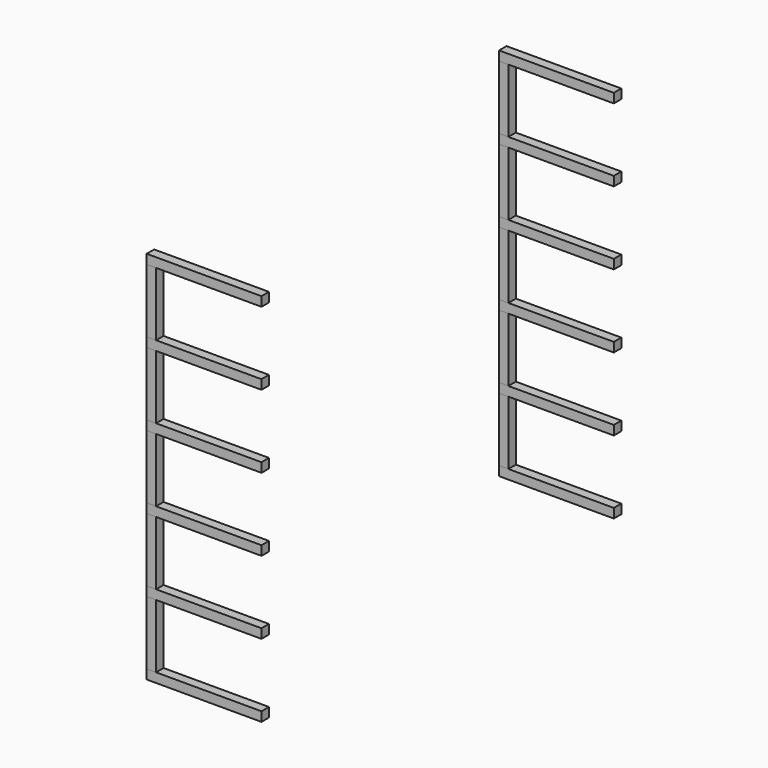
from build123d import *

# Parameters (mm, degrees)
F0_W     = 25.4
F0_H     = 25.4
F1_DEPTH = 311.15
F0_H_2   = 172.72
F2_DEPTH = 25.4
F3_DEPTH = 25.4
F4_DEPTH = 311.15


with BuildPart() as f1:
    # F0 (on Right) → F1 (new body)
    with BuildSketch(Plane.YZ):
        with Locations((-799.7573850555, 127.6102497262)):
            Rectangle(F0_W, F0_H)
    extrude(amount=F1_DEPTH)


with BuildPart() as f1b:
    # F0 (on Right) → F1, piece 2 (new body)
    with BuildSketch(Plane.YZ):
        with Locations((-799.7573850555, -466.7497502738)):
            Rectangle(F0_W, F0_H)
    extrude(amount=F1_DEPTH)


with BuildPart() as f1c:
    # F0 (on Right) → F1, piece 3 (new body)
    with BuildSketch(Plane.YZ):
        with Locations((-799.7573850555, 325.7302497262)):
            Rectangle(F0_W, F0_H)
    extrude(amount=F1_DEPTH)


with BuildPart() as f1d:
    # F0 (on Right) → F1, piece 4 (new body)
    with BuildSketch(Plane.YZ):
        with Locations((-799.7573850555, -268.6297502738)):
            Rectangle(F0_W, F0_H)
    extrude(amount=F1_DEPTH)


with BuildPart() as f1e:
    # F0 (on Right) → F1, piece 5 (new body)
    with BuildSketch(Plane.YZ):
        with Locations((-799.7573850555, -70.5097502738)):
            Rectangle(F0_W, F0_H)
    extrude(amount=F1_DEPTH)


with BuildPart() as f1f:
    # F0 (on Right) → F1, piece 6 (new body)
    with BuildSketch(Plane.YZ):
        with Locations((-799.7573850555, 523.8502497262)):
            Rectangle(F0_W, F0_H)
    extrude(amount=F1_DEPTH)


with BuildPart() as f2:
    # F0 (on Right) → F2 (new body)
    with BuildSketch(Plane.YZ):
        with Locations((-799.7573850555, -169.5697502738)):
            Rectangle(F0_W, F0_H_2)
    extrude(amount=F2_DEPTH)


with BuildPart() as f2b:
    # F0 (on Right) → F2, piece 2 (new body)
    with BuildSketch(Plane.YZ):
        with Locations((-799.7573850555, 226.6702497262)):
            Rectangle(F0_W, F0_H_2)
    extrude(amount=F2_DEPTH)


with BuildPart() as f2c:
    # F0 (on Right) → F2, piece 3 (new body)
    with BuildSketch(Plane.YZ):
        with Locations((-799.7573850555, 424.7902497262)):
            Rectangle(F0_W, F0_H_2)
    extrude(amount=F2_DEPTH)


with BuildPart() as f2d:
    # F0 (on Right) → F2, piece 4 (new body)
    with BuildSketch(Plane.YZ):
        with Locations((-799.7573850555, 28.5502497262)):
            Rectangle(F0_W, F0_H_2)
    extrude(amount=F2_DEPTH)


with BuildPart() as f2e:
    # F0 (on Right) → F2, piece 5 (new body)
    with BuildSketch(Plane.YZ):
        Polygon((-812.4573850555, -454.0497502738), (-787.0573850555, -454.0497502738), (-787.0573850555, -296.3315248489), (-787.0573850555, -281.3297502738), (-812.4573850555, -281.3297502738), (-812.4573850555, -296.3315248489), align=None)
    extrude(amount=F2_DEPTH)


with BuildPart() as f3:
    # F0 (on Right) → F3 (new body)
    with BuildSketch(Plane.YZ):
        Polygon((381.3426149445, -57.8097502738), (406.7426149445, -57.8097502738), (406.7426149445, 100.4313870019), (406.7426149445, 114.9102497262), (381.3426149445, 114.9102497262), align=None)
    extrude(amount=F3_DEPTH)


with BuildPart() as f3b:
    # F0 (on Right) → F3, piece 2 (new body)
    with BuildSketch(Plane.YZ):
        Polygon((381.3426149445, -255.9297502738), (406.7426149445, -255.9297502738), (406.7426149445, -83.2097502738), (393.4404167575, -83.2097502738), (381.3426149445, -83.2097502738), align=None)
    extrude(amount=F3_DEPTH)


with BuildPart() as f3c:
    # F0 (on Right) → F3, piece 3 (new body)
    with BuildSketch(Plane.YZ):
        with Locations((394.0426149445, 424.7902497262)):
            Rectangle(F0_W, F0_H_2)
    extrude(amount=F3_DEPTH)


with BuildPart() as f3d:
    # F0 (on Right) → F3, piece 4 (new body)
    with BuildSketch(Plane.YZ):
        Polygon((381.3426149445, -454.0497502738), (406.7426149445, -454.0497502738), (406.7426149445, -281.3297502738), (381.8395647449, -281.3297502738), (381.3426149445, -281.3297502738), align=None)
    extrude(amount=F3_DEPTH)


with BuildPart() as f3e:
    # F0 (on Right) → F3, piece 5 (new body)
    with BuildSketch(Plane.YZ):
        Polygon((381.3426149445, 140.3102497262), (406.7426149445, 140.3102497262), (406.7426149445, 313.0302497262), (395.5076758461, 313.0302497262), (381.3426149445, 313.0302497262), align=None)
    extrude(amount=F3_DEPTH)


with BuildPart() as f4:
    # F0 (on Right) → F4 (new body)
    with BuildSketch(Plane.YZ):
        Polygon((395.5076758461, 313.0302497262), (406.7426149445, 313.0302497262), (406.7426149445, 338.4302497262), (381.3426149445, 338.4302497262), (381.3426149445, 313.0302497262), align=None)
    extrude(amount=F4_DEPTH)


with BuildPart() as f4b:
    # F0 (on Right) → F4, piece 2 (new body)
    with BuildSketch(Plane.YZ):
        with Locations((394.0426149445, 523.8502497262)):
            Rectangle(F0_W, F0_H)
    extrude(amount=F4_DEPTH)


with BuildPart() as f4c:
    # F0 (on Right) → F4, piece 3 (new body)
    with BuildSketch(Plane.YZ):
        with Locations((394.0426149445, -466.7497502738)):
            Rectangle(F0_W, F0_H)
    extrude(amount=F4_DEPTH)


with BuildPart() as f4d:
    # F0 (on Right) → F4, piece 4 (new body)
    with BuildSketch(Plane.YZ):
        Polygon((381.8395647449, -281.3297502738), (406.7426149445, -281.3297502738), (406.7426149445, -255.9297502738), (381.3426149445, -255.9297502738), (381.3426149445, -281.3297502738), align=None)
    extrude(amount=F4_DEPTH)


with BuildPart() as f4e:
    # F0 (on Right) → F4, piece 5 (new body)
    with BuildSketch(Plane.YZ):
        with Locations((394.0426149445, 127.6102497262)):
            Rectangle(F0_W, F0_H)
    extrude(amount=F4_DEPTH)


with BuildPart() as f4f:
    # F0 (on Right) → F4, piece 6 (new body)
    with BuildSketch(Plane.YZ):
        Polygon((393.4404167575, -83.2097502738), (406.7426149445, -83.2097502738), (406.7426149445, -57.8097502738), (381.3426149445, -57.8097502738), (381.3426149445, -83.2097502738), align=None)
    extrude(amount=F4_DEPTH)


solid = Compound([f1.part, f1b.part, f1c.part, f1d.part, f1e.part, f1f.part, f2.part, f2b.part, f2c.part, f2d.part, f2e.part, f3.part, f3b.part, f3c.part, f3d.part, f3e.part, f4.part, f4b.part, f4c.part, f4d.part, f4e.part, f4f.part])
